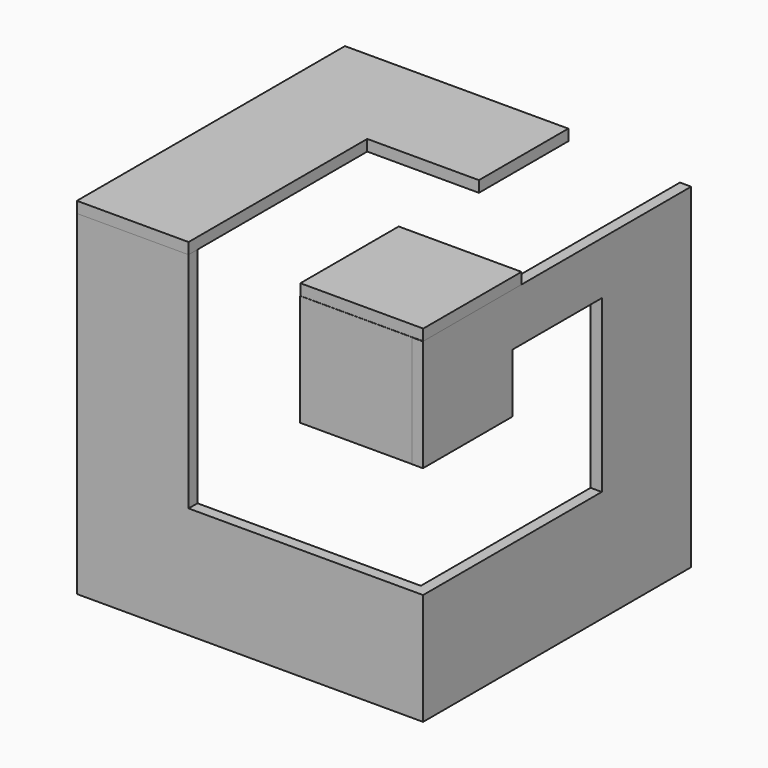
from build123d import *

# Parameters (mm, degrees)
F0_W     = 20
F0_H     = 40
F0_H_2   = 20
F0_W_2   = 40
F1_DEPTH = 2
F2_W     = 40
F2_H     = 20
F2_W_2   = 20
F2_W_3   = 20.0283188205
F2_H_2   = 9.4384654047
F3_DEPTH = 2
F4_W     = 20
F4_H     = 40
F4_H_2   = 20
F5_DEPTH = 2
F4_W_2   = 22
F4_H_3   = 22


with BuildPart() as f1:
    # F0 (on Front) → F1 (new body)
    with BuildSketch(Plane.XZ):
        with Locations((-35.8879165724, 7.8213110747)):
            Rectangle(F0_W, F0_H)
        with Locations((-35.8879165724, -22.1786889253)):
            Rectangle(F0_W, F0_H_2)
        with Locations((-5.8879165724, -22.1786889253)):
            Rectangle(F0_W_2, F0_H_2)
    extrude(amount=F1_DEPTH)

    # F2 (on face) → F3 (join)
    with BuildSketch(Plane.YZ.offset(14.1120834276)):
        with Locations((18, -22.1786889253)):
            Rectangle(F2_W, F2_H)
        with Locations((48, -22.1786889253)):
            Rectangle(F2_W_2, F2_H)
        Polygon((38, 18.38284567), (38, -12.1786889253), (58, -12.1786889253), (58, 27.8213110747), (38, 27.8213110747), align=None)
        with Locations((27.9858405897, 23.1020783723)):
            Rectangle(F2_W_3, F2_H_2)
        Polygon((17.9716811795, 7.8213110747), (17.9716811795, 18.38284567), (17.9716811795, 27.8213110747), (-2.0283188205, 27.8213110747), (-2.0283188205, 7.8213110747), align=None)
    extrude(amount=F3_DEPTH)


with BuildPart() as f1b:
    # F0 (on Front) → F1, piece 2 (new body)
    with BuildSketch(Plane.XZ):
        with Locations((4.1120834276, 17.8213110747)):
            Rectangle(F0_W, F0_H_2)
    extrude(amount=F1_DEPTH)


with BuildPart() as f5:
    # F4 (on face) → F5 (new body)
    with BuildSketch(Plane.XY.offset(27.8213110747)):
        with Locations((-35.8879165724, 18)):
            Rectangle(F4_W, F4_H)
        with Locations((-35.8879165724, 48)):
            Rectangle(F4_W, F4_H_2)
        with Locations((-15.8879165724, 48)):
            Rectangle(F4_W, F4_H_2)
    extrude(amount=F5_DEPTH)


with BuildPart() as f5b:
    # F4 (on face) → F5, piece 2 (new body)
    with BuildSketch(Plane.XY.offset(27.8213110747)):
        with Locations((5.1120834276, 9.0354546569)):
            Rectangle(F4_W_2, F4_H_3)
    extrude(amount=F5_DEPTH)


solid = Compound([f1.part, f1b.part, f5.part, f5b.part])
